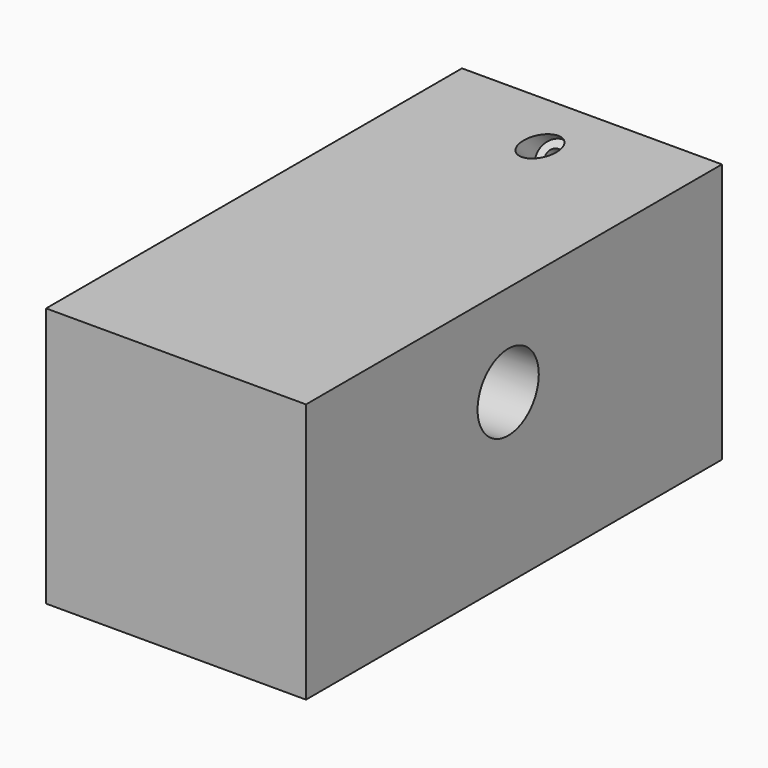
from build123d import *

# Parameters (mm, degrees)
F0_W          = 101.6
F0_H          = 101.6
F1_DEPTH      = 203.2
F4_R          = 3.175
F5_DEPTH      = 89.8035612107
F4_R_2        = 6.35
F6_DEPTH      = 9.525
F6_DEPTH_BACK = 125.724585695
F8_R          = 14.9564756193
F9_DEPTH      = 25.4


# Not quite as in the source:
# - a pattern or mirror of a feature is missing from the dataset's text; its kind, count and spacing are read off the source's solid


with BuildPart() as f1:
    # F0 (on Front) → F1 (new body)
    with BuildSketch(Plane.XZ):
        with Locations((50.8, 50.8)):
            Rectangle(F0_W, F0_H)
    extrude(amount=F1_DEPTH)

    # F4 (on line) → F5 (cut, through all)
    with BuildSketch(Plane(origin=(0, -63.5, 63.5), x_dir=(-1, 0, 0), z_dir=(0, 0.7071067812, -0.7071067812))):
        with Locations((-50.8, 53.8815367264)):
            Circle(F4_R)
    f5 = extrude(amount=F5_DEPTH, mode=Mode.SUBTRACT)

    # F5_copies: F5 across plane
    add(f5.mirror(Plane(origin=(0, 1.2e-05, 50.799992), x_dir=(-1, 0, 0), z_dir=(0, 0, -1))), mode=Mode.SUBTRACT)

    # F4 (on line) → F6 (cut, two sides)
    with BuildSketch(Plane(origin=(0, -63.5, 63.5), x_dir=(-1, 0, 0), z_dir=(0, 0.7071067812, -0.7071067812))) as f6_sk:
        with Locations((-50.8, 53.8815367264)):
            Circle(F4_R_2)
        with Locations((-50.8, 53.8815367264)):
            Circle(F4_R, mode=Mode.SUBTRACT)
        with Locations((-50.8, 53.8815367264)):
            Circle(F4_R)
    f6 = extrude(amount=F6_DEPTH, mode=Mode.SUBTRACT) + extrude(f6_sk.sketch, amount=-F6_DEPTH_BACK, mode=Mode.SUBTRACT)

    # F6_copies: F6 across plane
    add(f6.mirror(Plane(origin=(0, 2.8e-05, 50.79997), x_dir=(0, -1, 1e-06), z_dir=(0, -1e-06, -1))), mode=Mode.SUBTRACT)

    # F8 (on face) → F9 (cut)
    with BuildSketch(Plane.YZ.offset(101.6)):
        with Locations((-104.4293493032, 65.6716227531)):
            Circle(F8_R)
    extrude(amount=-F9_DEPTH, mode=Mode.SUBTRACT)


solid = f1.part
